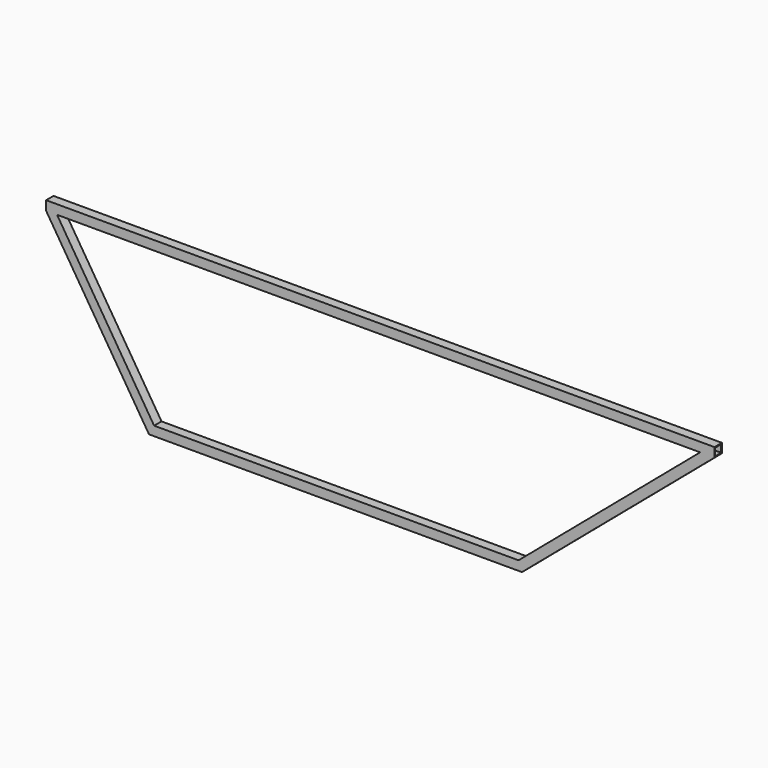
from build123d import *

# Parameters (mm, degrees)
F1_DEPTH      = 7.9375
F2_W          = 12.6746
F2_H          = 12.6746
F3_DEPTH      = 1143.001
F3_DEPTH_BACK = 1751


# Not quite as in the source:
# - an extrude ends at something that could not be found from the text; its depth is read off the source's solid


with BuildPart() as f1:
    # F0 (on Front) → F1 (new body, symmetric)
    with BuildSketch(Plane.XZ):
        Polygon((242.2783725209, -287.3375), (571.5, -7.9375), (571.5, 7.9375), (-571.5, 7.9375), (-571.5, -7.9375), (-395.523637951, -287.3375), align=None)
        Polygon((-386.7609312492, -271.4625), (-552.7386363636, -7.9375), (546.9659090909, -7.9375), (236.4500559004, -271.4625), align=None, mode=Mode.SUBTRACT)
    extrude(amount=F1_DEPTH, both=True)

    # F2 (on face) → F3 (cut, two sides)
    with BuildSketch(Plane(origin=(-571.5, 0, 0), x_dir=(0, -1, 0), z_dir=(-1, 0, 0))) as f3_sk:
        Rectangle(F2_W, F2_H)
    extrude(amount=-F3_DEPTH, mode=Mode.SUBTRACT)
    extrude(f3_sk.sketch, amount=F3_DEPTH_BACK, mode=Mode.SUBTRACT)


solid = f1.part
